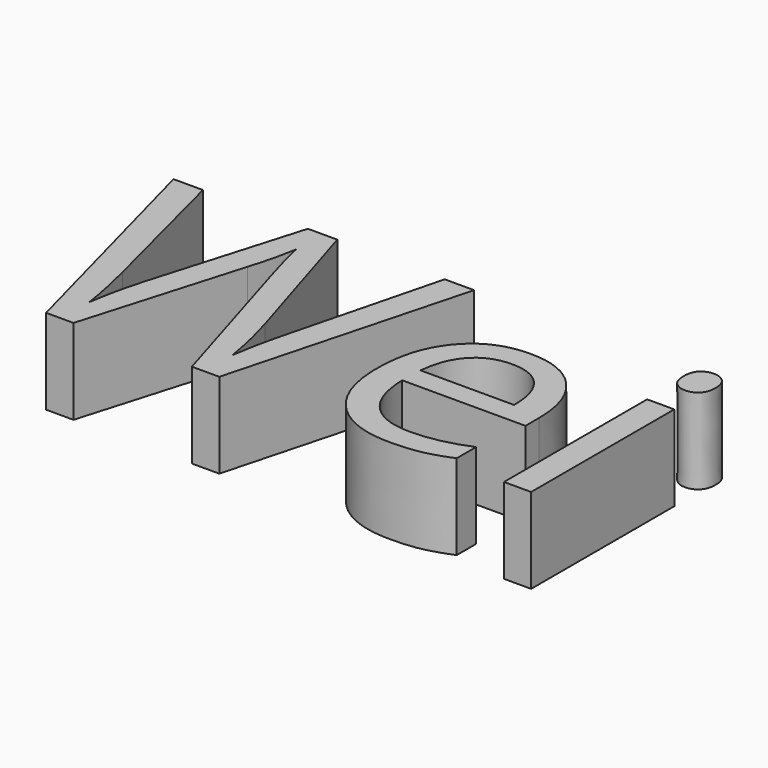
from build123d import *

# Parameters (mm, degrees)
F0_TEXT_SIZE = 99.5489096062
F1_DEPTH     = 25.4


# Not quite as in the source:
# - Text() gives the source's letters only with a copy of the font that has no kerning and outlines rounded to 1/6400 em; it was checked with that copy


with BuildPart() as f1:
    # F0 (on Top) → F1 (new body)
    with BuildSketch(Plane.XY):
        with Locations((-64.1759335995, -11.1189559102)):
            Text('Wei', F0_TEXT_SIZE, font='Open Sans', text_align=(TextAlign.LEFT, TextAlign.BOTTOM))
    extrude(amount=F1_DEPTH)


solid = f1.part
